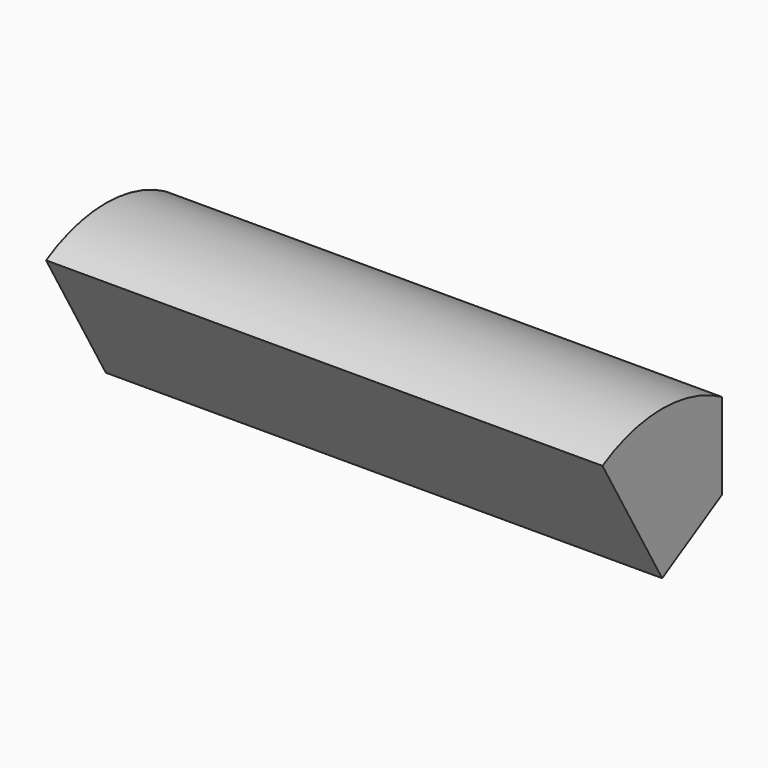
from build123d import *

# Parameters (mm, degrees)
F1_DEPTH = 112.7125


# Not quite as in the source:
# - a feature of the source that left no trace in its solid (it failed there, or was rolled back) is left out


with BuildPart() as f1:
    # F0 (on Right) → F1 (new body, symmetric)
    with BuildSketch(Plane.YZ):
        with BuildLine():
            Line((-60.4918744543, 34.925), (-30.2459372272, -17.4625))
            Line((-30.2459372272, -17.4625), (0, 0))
            Line((0, 0), (0, 34.925))
            ThreePointArc((0, 34.925), (-30.2459372272, 43.0293744543), (-60.4918744543, 34.925))
        make_face()
    extrude(amount=F1_DEPTH, both=True)


solid = f1.part
